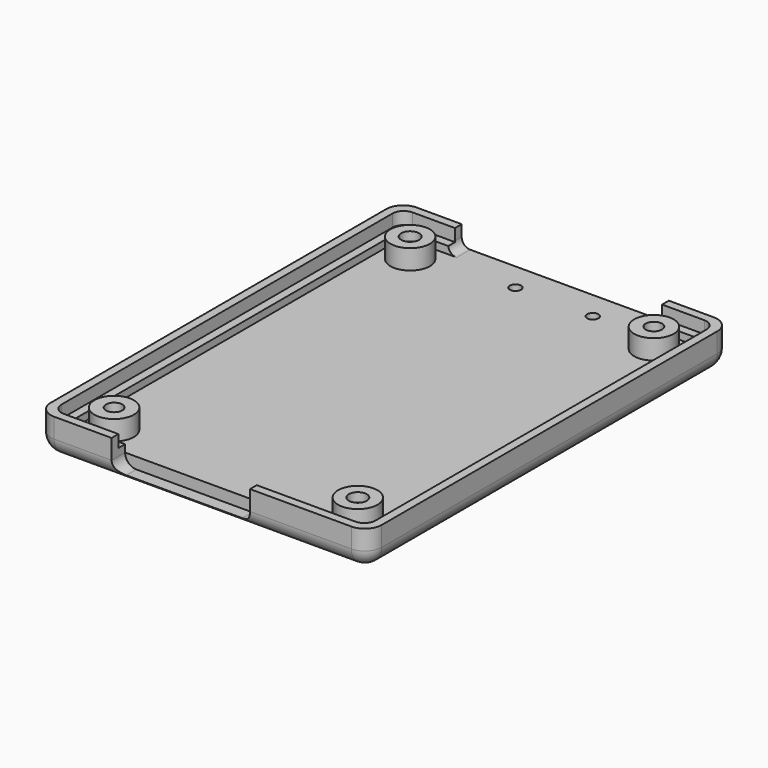
from build123d import *

# Parameters (mm, degrees)
F0_W          = 58.8
F0_H          = 80.5
F1_DEPTH      = 6.5
F2_W          = 52.8
F2_H          = 74.5
F3_DEPTH      = 3.5
F5_R          = 3.5
F6_DEPTH      = 3.5
F8_R          = 1.45
F10_R         = 1.45
F11_DEPTH     = 6.501
F9_R          = 1.6
F7_R          = 1.6
F12_DEPTH     = 1.6
F13_W         = 36.8
F13_H         = 3
F14_DEPTH     = 3.5
F15_W         = 24.6
F15_H         = 3
F16_DEPTH     = 5.5
F19_DEPTH     = 2.2
F20_R         = 1
F21_DEPTH     = 6.501
F22_T1_DEPTH  = 11
F22_T3_DEPTH  = 52.8
F22_T5_DEPTH  = 74.5
F22_S9_W      = 3
F22_S9_H      = 3
F22_T10_DEPTH = 3
F22_S15_W     = 3
F22_S15_H     = 3
F22_T16_DEPTH = 3
F22_S21_W     = 3
F22_S21_H     = 3
F22_T22_DEPTH = 3
F22_S27_W     = 3
F22_S27_H     = 3
F22_T28_DEPTH = 3
F24_R         = 2
F25_R         = 1.5
F26_R         = 2
F27_R         = 2.75
F28_DEPTH     = 1.6


# Not quite as in the source:
# - a fillet or chamfer that OpenCascade refuses, or shapes differently, is made with other operations: its cross-section is extruded or revolved along the edge and cut away or added
# - a feature of the source that left no trace in its solid (it failed there, or was rolled back) is left out


with BuildPart() as f1:
    # F0 (on Top) → F1 (new body)
    with BuildSketch(Plane.XY):
        with Locations((29.4, 40.25)):
            Rectangle(F0_W, F0_H)
    extrude(amount=F1_DEPTH)

    # F2 (on face) → F3 (cut)
    with BuildSketch(Plane.XY.offset(6.5)):
        with Locations((29.4, 40.25)):
            Rectangle(F2_W, F2_H)
    extrude(amount=-F3_DEPTH, mode=Mode.SUBTRACT)

    # F5 (on face) → F6 (join)
    with BuildSketch(Plane.XY.offset(3)):
        with Locations((7.75, 7.375)):
            Circle(F5_R)
        with Locations((7.75, 73.125)):
            Circle(F5_R)
        with Locations((51.05, 73.125)):
            Circle(F5_R)
        with Locations((51.05, 7.375)):
            Circle(F5_R)
    extrude(amount=F6_DEPTH)

    # F8 (on face) + F10 (on face) → F11 (cut, through all)
    with BuildSketch(Plane.XY.offset(6.5)):
        with Locations((51.05, 73.125)):
            Circle(F8_R)
    with BuildSketch(Plane.XY.offset(6.5)):
        with Locations((7.75, 7.375)):
            Circle(F10_R)
    extrude(amount=-F11_DEPTH, mode=Mode.SUBTRACT)

    # F9 (on face) + F7 (on face) → F12 (cut)
    with BuildSketch(Plane.XY.offset(6.5)):
        with Locations((7.75, 73.125)):
            Circle(F9_R)
    with BuildSketch(Plane.XY.offset(6.5)):
        with Locations((51.05, 7.375)):
            Circle(F7_R)
    extrude(amount=-F12_DEPTH, mode=Mode.SUBTRACT)

    # F13 (on face) → F14 (cut)
    with BuildSketch(Plane.XY.offset(6.5)):
        with Locations((29.4, 79)):
            Rectangle(F13_W, F13_H)
    extrude(amount=-F14_DEPTH, mode=Mode.SUBTRACT)

    # F15 (on face) → F16 (cut)
    with BuildSketch(Plane.XY.offset(6.5)):
        with Locations((25.5, 1.5)):
            Rectangle(F15_W, F15_H)
    extrude(amount=-F16_DEPTH, mode=Mode.SUBTRACT)

    # F17 (on face) + F18 (on face) → F19 (cut)
    with BuildSketch(Plane.XY.offset(6.5)):
        Polygon((47.8, 79), (47.8, 77.5), (55.8, 77.5), (55.8, 3), (37.8, 3), (37.8, 1.5), (57.3, 1.5), (57.3, 79), align=None)
    with BuildSketch(Plane.XY.offset(6.5)):
        Polygon((1.5, 1.5), (13.2, 1.5), (13.2, 3), (3, 3), (3, 77.5), (11, 77.5), (11, 79), (1.5, 79), align=None)
    extrude(amount=-F19_DEPTH, mode=Mode.SUBTRACT)

    # F20 (on face) → F21 (cut, through all)
    with BuildSketch(Plane(origin=(0, 0, 0), x_dir=(1, 0, 0), z_dir=(0, 0, -1))):
        with Locations((39.3, -5)):
            Circle(F20_R)
        with Locations((38.3, -75.5)):
            Circle(F20_R)
        with Locations((24.55, -75.5)):
            Circle(F20_R)
    extrude(amount=-F21_DEPTH, mode=Mode.SUBTRACT)

    # F22: fillet of radius 3 on 8 edges, made by hand

    # F22_s2 → F22_t1 (cut)
    with BuildSketch(Plane.XY.offset(3)):
        with BuildLine():
            ThreePointArc((0, 3), (0.8786796564, 0.8786796564), (3, 0))
            Line((3, 0), (0, 0))
            Line((0, 0), (0, 3))
        make_face()
        with BuildLine():
            ThreePointArc((55.8, 0), (57.9213203436, 0.8786796564), (58.8, 3))
            Line((58.8, 3), (58.8, 0))
            Line((58.8, 0), (55.8, 0))
        make_face()
        with BuildLine():
            ThreePointArc((0, 77.5), (0.8786796564, 79.6213203436), (3, 80.5))
            Line((3, 80.5), (0, 80.5))
            Line((0, 80.5), (0, 77.5))
        make_face()
        with BuildLine():
            ThreePointArc((55.8, 80.5), (57.9213203436, 79.6213203436), (58.8, 77.5))
            Line((58.8, 77.5), (58.8, 80.5))
            Line((58.8, 80.5), (55.8, 80.5))
        make_face()
    extrude(amount=F22_T1_DEPTH, mode=Mode.SUBTRACT)

    # F22_s4 → F22_t3 (cut)
    with BuildSketch(Plane.YZ.offset(3)):
        with BuildLine():
            ThreePointArc((0, 3), (0.8786796564, 0.8786796564), (3, 0))
            Line((3, 0), (0, 0))
            Line((0, 0), (0, 3))
        make_face()
        with BuildLine():
            ThreePointArc((80.5, 3), (79.6213203436, 0.8786796564), (77.5, 0))
            Line((77.5, 0), (80.5, 0))
            Line((80.5, 0), (80.5, 3))
        make_face()
    extrude(amount=F22_T3_DEPTH, mode=Mode.SUBTRACT)

    # F22_s6 → F22_t5 (cut)
    with BuildSketch(Plane.XZ.offset(-77.5)):
        with BuildLine():
            ThreePointArc((0, 3), (0.8786796564, 0.8786796564), (3, 0))
            Line((3, 0), (0, 0))
            Line((0, 0), (0, 3))
        make_face()
        with BuildLine():
            ThreePointArc((55.8, 0), (57.9213203436, 0.8786796564), (58.8, 3))
            Line((58.8, 3), (58.8, 0))
            Line((58.8, 0), (55.8, 0))
        make_face()
    extrude(amount=F22_T5_DEPTH, mode=Mode.SUBTRACT)


with BuildPart() as f22_tool8:
    # F22_s9 → F22_t10 (new body)
    with BuildSketch(Plane.YZ.offset(3)):
        with Locations((1.5, 1.5)):
            Rectangle(F22_S9_W, F22_S9_H)
    extrude(amount=-F22_T10_DEPTH)

    # F22_s11 → F22_t12 (revolve, cut)
    with BuildSketch(Plane(origin=(3, 3, 3), x_dir=(0, 0.7071067812, 0.7071067812), z_dir=(0, -0.7071067812, 0.7071067812))):
        with BuildLine():
            ThreePointArc((0, -3), (3, 0), (0, 3))
            Line((0, 3), (0, -3))
        make_face()
    revolve(axis=Axis((3, 3, 3), (-1, 0, 0)), mode=Mode.SUBTRACT)


with BuildPart() as f1_1:
    add(f1.part)

    # F22_t7: cut F22_tool8
    add(f22_tool8.part, mode=Mode.SUBTRACT)


with BuildPart() as f22_tool14:
    # F22_s15 → F22_t16 (new body)
    with BuildSketch(Plane.YZ.offset(55.8)):
        with Locations((1.5, 1.5)):
            Rectangle(F22_S15_W, F22_S15_H)
    extrude(amount=F22_T16_DEPTH)

    # F22_s17 → F22_t18 (revolve, cut)
    with BuildSketch(Plane(origin=(55.8, 3, 3), x_dir=(0, 0.7071067812, 0.7071067812), z_dir=(0, 0.7071067812, -0.7071067812))):
        with BuildLine():
            ThreePointArc((0, -3), (3, 0), (0, 3))
            Line((0, 3), (0, -3))
        make_face()
    revolve(axis=Axis((55.8, 3, 3), (1, 0, 0)), mode=Mode.SUBTRACT)


with BuildPart() as f1_2:
    add(f1_1.part)

    # F22_t13: cut F22_tool14
    add(f22_tool14.part, mode=Mode.SUBTRACT)


with BuildPart() as f22_tool20:
    # F22_s21 → F22_t22 (new body)
    with BuildSketch(Plane.YZ.offset(3)):
        with Locations((79, 1.5)):
            Rectangle(F22_S21_W, F22_S21_H)
    extrude(amount=-F22_T22_DEPTH)

    # F22_s23 → F22_t24 (revolve, cut)
    with BuildSketch(Plane(origin=(3, 77.5, 3), x_dir=(0, -0.7071067812, 0.7071067812), z_dir=(0, -0.7071067812, -0.7071067812))):
        with BuildLine():
            ThreePointArc((0, -3), (3, 0), (0, 3))
            Line((0, 3), (0, -3))
        make_face()
    revolve(axis=Axis((3, 77.5, 3), (-1, 0, 0)), mode=Mode.SUBTRACT)


with BuildPart() as f1_3:
    add(f1_2.part)

    # F22_t19: cut F22_tool20
    add(f22_tool20.part, mode=Mode.SUBTRACT)


with BuildPart() as f22_tool26:
    # F22_s27 → F22_t28 (new body)
    with BuildSketch(Plane.XZ.offset(-77.5)):
        with Locations((57.3, 1.5)):
            Rectangle(F22_S27_W, F22_S27_H)
    extrude(amount=-F22_T28_DEPTH)

    # F22_s29 → F22_t30 (revolve, cut)
    with BuildSketch(Plane(origin=(55.8, 77.5, 3), x_dir=(-0.7071067812, 0, 0.7071067812), z_dir=(-0.7071067812, 0, -0.7071067812))):
        with BuildLine():
            ThreePointArc((0, -3), (3, 0), (0, 3))
            Line((0, 3), (0, -3))
        make_face()
    revolve(axis=Axis((55.8, 77.5, 3), (0, 1, 0)), mode=Mode.SUBTRACT)


with BuildPart() as f1_4:
    add(f1_3.part)

    # F22_t25: cut F22_tool26
    add(f22_tool26.part, mode=Mode.SUBTRACT)

    # F24
    f24_edges = [f1_4.edges().sort_by_distance(p)[0] for p in [
        (57.3, 79, 5.4),
        (57.3, 1.5, 5.4),
        (1.5, 1.5, 5.4),
        (1.5, 79, 5.4),
    ]]
    fillet(f24_edges, radius=F24_R)

    # F25#2 (call 1 of 2: OpenCascade refuses the feature's edges together)
    f25_2_edges = [f1_4.edges().sort_by_distance(p)[0] for p in [
        (47.8, 79, 3),
    ]]
    fillet(f25_2_edges, radius=F25_R)

    # F25 (call 2 of 2)
    f25_edges = [f1_4.edges().sort_by_distance(p)[0] for p in [
        (11, 79, 3),
    ]]
    fillet(f25_edges, radius=F25_R)

    # F26
    f26_edges = [f1_4.edges().sort_by_distance(p)[0] for p in [
        (13.2, 1.881966, 1),
        (37.8, 1.881966, 1),
    ]]
    fillet(f26_edges, radius=F26_R)

    # F27 (on face) → F28 (cut)
    with BuildSketch(Plane(origin=(0, 0, 0), x_dir=(1, 0, 0), z_dir=(0, 0, -1))):
        with Locations((51.05, -73.125)):
            Circle(F27_R)
        with Locations((7.75, -7.375)):
            Circle(F27_R)
    extrude(amount=-F28_DEPTH, mode=Mode.SUBTRACT)


solid = f1_4.part
